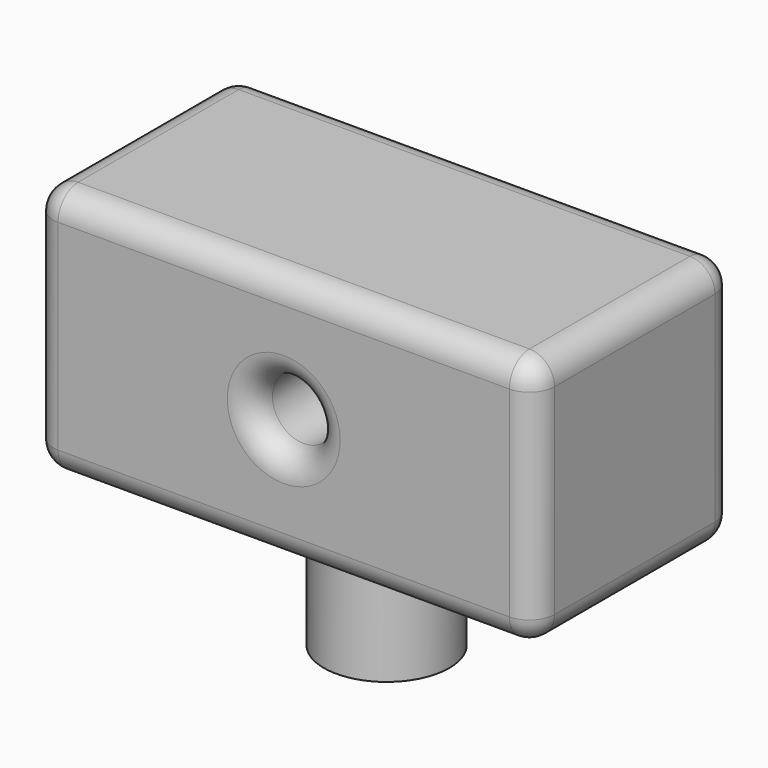
from build123d import *

# Parameters (mm, degrees)
F0_W           = 101.6
F0_H           = 50.8
F1_DEPTH       = 50.8
F3_D           = 12.7
F3_CBORE_D     = 25.4
F3_CBORE_DEPTH = 6.35
F5_R           = 12.7
F6_DEPTH       = 25.4
F7_R           = 5.08


with BuildPart() as f1:
    # F0 (on Top) → F1 (new body)
    with BuildSketch(Plane.XY):
        with Locations((50.8, 25.4)):
            Rectangle(F0_W, F0_H)
    extrude(amount=F1_DEPTH)

    # F3 (through all)
    with Locations(Plane(origin=(0, 50.8, 0), x_dir=(-1, 0, 0), z_dir=(0, 1, 0))):
        with Locations((-50.8, 25.4)):
            CounterBoreHole(F3_D / 2, F3_CBORE_D / 2, F3_CBORE_DEPTH)

    # F5 (on offset) → F6 (join, through all)
    with BuildSketch(Plane(origin=(0, 0, -25.4), x_dir=(1, 0, 0), z_dir=(0, 0, -1))):
        with Locations((50.8, -26.0627344251)):
            Circle(F5_R)
    extrude(amount=-F6_DEPTH)

    # F7
    f7_edges = [f1.edges().sort_by_distance(p)[0] for p in [
        (101.6, 0, 25.4),
        (101.6, 50.8, 25.4),
        (101.6, 25.4, 0),
        (101.6, 25.4, 50.8),
        (0, 50.8, 25.4),
        (0, 0, 25.4),
        (0, 25.4, 0),
        (0, 25.4, 50.8),
        (50.8, 0, 50.8),
        (50.8, 50.8, 50.8),
        (50.8, 0, 0),
        (57.15, 0, 25.4),
        (50.8, 50.8, 0),
    ]]
    fillet(f7_edges, radius=F7_R)


solid = f1.part
